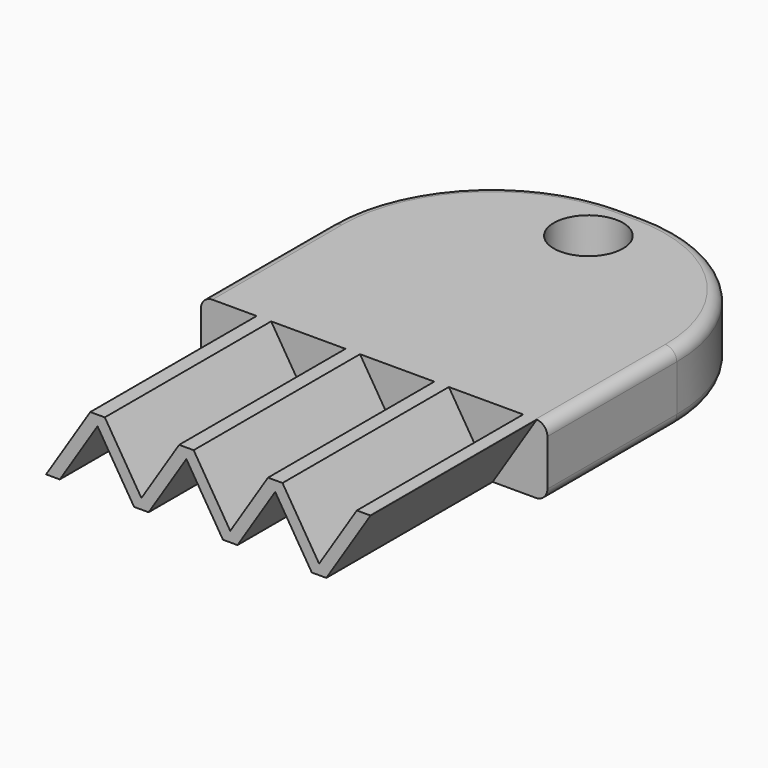
from build123d import *

# Parameters (mm, degrees)
F0_R     = 3
F1_DEPTH = 6
F3_R     = 1
F5_DEPTH = 18


with BuildPart() as f1:
    # F0 (on Top) → F1 (new body)
    with BuildSketch(Plane.XY):
        with BuildLine():
            Line((-15, -14), (15, -14))
            Line((15, -14), (15, 0))
            ThreePointArc((15, 0), (10.8994949366, 9.8994949366), (1, 14))
            Line((1, 14), (-1, 14))
            ThreePointArc((-1, 14), (-10.8994949366, 9.8994949366), (-15, 0))
            Line((-15, 0), (-15, -14))
        make_face()
        with Locations((0, 9.1889705509)):
            Circle(F0_R, mode=Mode.SUBTRACT)
    extrude(amount=F1_DEPTH)

    # F3
    f3_edges = [f1.edges().sort_by_distance(p)[0] for p in [
        (-10.899495, 9.899495, 6),
        (10.899495, 9.899495, 6),
        (-15, -7, 6),
        (15, -7, 6),
        (-15, -7, 0),
        (-10.899495, 9.899495, 0),
        (10.899495, 9.899495, 0),
        (15, -7, 0),
    ]]
    fillet(f3_edges, radius=F3_R)

    # F4 (on face) → F5 (join)
    with BuildSketch(Plane.XZ.offset(14)):
        with BuildLine():
            Line((-10.1717880173, 6), (-14, 0))
            Line((-14, 0), (-12.8137921418, 0))
            Line((-12.8137921418, 0), (-9.5468121047, 5.120374815))
            Line((-9.5468121047, 5.120374815), (-6.3790735405, 0))
            Line((-6.3790735405, 0), (-5.122384561, 0))
            Line((-5.122384561, 0), (-1.8554045239, 5.120374815))
            Line((-1.8554045239, 5.120374815), (1.3123340403, 0))
            Line((1.3123340403, 0), (2.5690230199, 0))
            Line((2.5690230199, 0), (5.836003057, 5.120374815))
            Line((5.836003057, 5.120374815), (9.0037416211, 0))
            Line((9.0037416211, 0), (10.2604306007, 0))
            Line((10.2604306007, 0), (14.0862641777, 5.9962722979))
            ThreePointArc((14.0862641777, 5.9962722979), (14.043172341, 5.9990676398), (14, 6))
            Line((14, 6), (12.9024347251, 6))
            Line((12.9024347251, 6), (9.635454688, 0.879625185))
            Line((9.635454688, 0.879625185), (6.4677161239, 6))
            Line((6.4677161239, 6), (5.2110271443, 6))
            Line((5.2110271443, 6), (1.9440471072, 0.879625185))
            Line((1.9440471072, 0.879625185), (-1.223691457, 6))
            Line((-1.223691457, 6), (-2.4803804365, 6))
            Line((-2.4803804365, 6), (-5.7473604736, 0.879625185))
            Line((-5.7473604736, 0.879625185), (-8.9150990378, 6))
            Line((-8.9150990378, 6), (-10.1717880173, 6))
        make_face()
    extrude(amount=F5_DEPTH)


solid = f1.part
